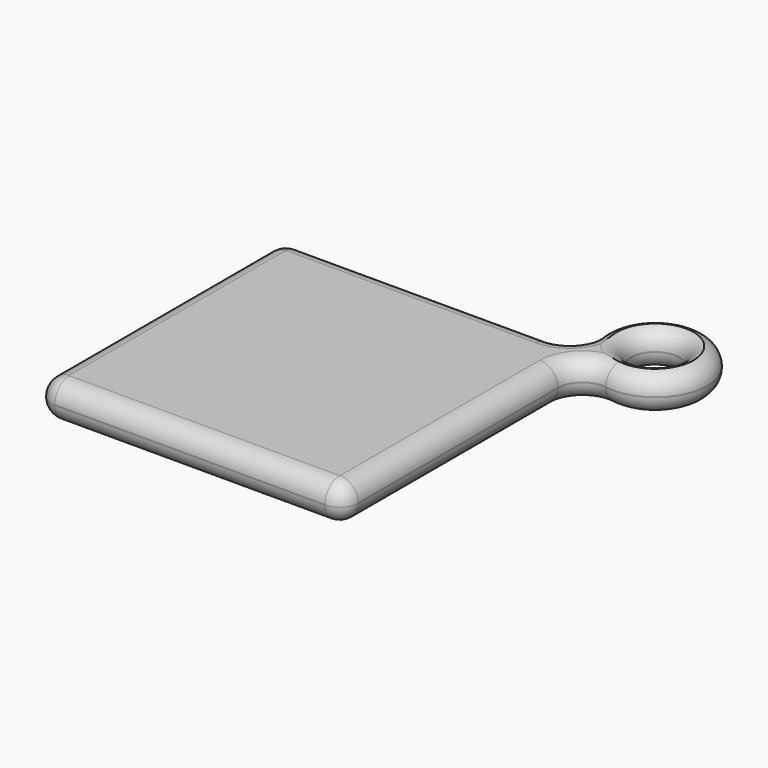
from build123d import *

# Parameters (mm, degrees)
F0_R         = 2
F1_DEPTH     = 3
F2_T1_DEPTH  = 20.3370084506
F2_T3_DEPTH  = 21.9980686292
F2_T5_DEPTH  = 21.9980686292
F2_T7_DEPTH  = 20.3370084506
F2_S11_W     = 1.6515022539
F2_S11_H     = 1.6515022539
F2_T12_DEPTH = 1.651502254
F2_S17_W     = 1.6515022539
F2_S17_H     = 1.6515022539
F2_T18_DEPTH = 1.651502254
F2_S23_W     = 1.6515022539
F2_S23_H     = 1.6515022539
F2_T24_DEPTH = 1.651502254
F2_S29_W     = 1.6515022539
F2_S29_H     = 1.6515022539
F2_T30_DEPTH = 1.651502254
F2_S35_W     = 1.6515022539
F2_S35_H     = 1.6515022539
F2_T36_DEPTH = 1.651502254
F2_S41_W     = 1.6515022539
F2_S41_H     = 1.6515022539
F2_T42_DEPTH = 1.651502254
F2_T46_ANGLE = 99.2178445956
F2_T48_ANGLE = 288.4356891912
F2_T50_ANGLE = 99.2178445956
F2_T54_ANGLE = 99.2178445956
F2_T56_ANGLE = 288.4356891912
F2_T58_ANGLE = 99.2178445956


# Not quite as in the source:
# - a fillet or chamfer that OpenCascade refuses, or shapes differently, is made with other operations: its cross-section is extruded or revolved along the edge and cut away or added


with BuildPart() as f1:
    # F0 (on Top) → F1 (new body)
    with BuildSketch(Plane.XY):
        with BuildLine():
            Line((0, 25), (0, 0))
            Line((0, 0), (25, 0))
            Line((25, 0), (25, 21.837974136))
            ThreePointArc((25, 21.837974136), (25.7039973924, 23.3612525876), (27.320377241, 23.8121469814))
            ThreePointArc((27.320377241, 23.8121469814), (31.7765520504, 26.0666985205), (31, 31))
            ThreePointArc((31, 31), (26.0666985205, 31.7765520504), (23.8121469814, 27.320377241))
            ThreePointArc((23.8121469814, 27.320377241), (23.3612525876, 25.7039973924), (21.837974136, 25))
            Line((21.837974136, 25), (0, 25))
        make_face()
        with Locations((28, 28)):
            Circle(F0_R, mode=Mode.SUBTRACT)
    extrude(amount=F1_DEPTH)

    # F2: fillet of radius 1.5 on 19 edges, made by hand

    # F2_s2 → F2_t1 (cut)
    with BuildSketch(Plane.YZ.offset(1.5009656854)):
        with BuildLine():
            ThreePointArc((25.0004, 1.4990343146), (24.5606601718, 2.5606601718), (23.4990343146, 3.0004))
            Line((23.4990343146, 3.0004), (23.4990343146, 3.1505365685))
            ThreePointArc((23.4990343146, 3.1505365685), (24.2495171573, 3.1501365685), (25, 3.1501365685))
            Line((25, 3.1501365685), (25.1501365685, 3))
            ThreePointArc((25.1501365685, 3), (25.1501365685, 2.2495171573), (25.1505365685, 1.4990343146))
            Line((25.1505365685, 1.4990343146), (25.0004, 1.4990343146))
        make_face()
        with BuildLine():
            ThreePointArc((25.0004, 1.5009656854), (24.5606601718, 0.4393398282), (23.4990343146, -0.0004))
            Line((23.4990343146, -0.0004), (23.4990343146, -0.1505365685))
            ThreePointArc((23.4990343146, -0.1505365685), (24.2495171573, -0.1501365685), (25, -0.1501365685))
            Line((25, -0.1501365685), (25.1501365685, 0))
            ThreePointArc((25.1501365685, 0), (25.1501365685, 0.7504828427), (25.1505365685, 1.5009656854))
            Line((25.1505365685, 1.5009656854), (25.0004, 1.5009656854))
        make_face()
    extrude(amount=F2_T1_DEPTH, mode=Mode.SUBTRACT)

    # F2_s4 → F2_t3 (cut)
    with BuildSketch(Plane.XZ.offset(-23.4990343146)):
        with BuildLine():
            ThreePointArc((1.5009656854, 3.0004), (0.4393398282, 2.5606601718), (-0.0004, 1.4990343146))
            Line((-0.0004, 1.4990343146), (-0.1505365685, 1.4990343146))
            ThreePointArc((-0.1505365685, 1.4990343146), (-0.1501365685, 2.2495171573), (-0.1501365685, 3))
            Line((-0.1501365685, 3), (0, 3.1501365685))
            ThreePointArc((0, 3.1501365685), (0.7504828427, 3.1501365685), (1.5009656854, 3.1505365685))
            Line((1.5009656854, 3.1505365685), (1.5009656854, 3.0004))
        make_face()
        with BuildLine():
            ThreePointArc((1.5009656854, -0.0004), (0.4393398282, 0.4393398282), (-0.0004, 1.5009656854))
            Line((-0.0004, 1.5009656854), (-0.1505365685, 1.5009656854))
            ThreePointArc((-0.1505365685, 1.5009656854), (-0.1501365685, 0.7504828427), (-0.1501365685, 0))
            Line((-0.1501365685, 0), (0, -0.1501365685))
            ThreePointArc((0, -0.1501365685), (0.7504828427, -0.1501365685), (1.5009656854, -0.1505365685))
            Line((1.5009656854, -0.1505365685), (1.5009656854, -0.0004))
        make_face()
    extrude(amount=F2_T3_DEPTH, mode=Mode.SUBTRACT)

    # F2_s6 → F2_t5 (cut)
    with BuildSketch(Plane.YZ.offset(1.5009656854)):
        with BuildLine():
            ThreePointArc((1.5009656854, 3.0004), (0.4393398282, 2.5606601718), (-0.0004, 1.4990343146))
            Line((-0.0004, 1.4990343146), (-0.1505365685, 1.4990343146))
            ThreePointArc((-0.1505365685, 1.4990343146), (-0.1501365685, 2.2495171573), (-0.1501365685, 3))
            Line((-0.1501365685, 3), (0, 3.1501365685))
            ThreePointArc((0, 3.1501365685), (0.7504828427, 3.1501365685), (1.5009656854, 3.1505365685))
            Line((1.5009656854, 3.1505365685), (1.5009656854, 3.0004))
        make_face()
        with BuildLine():
            ThreePointArc((-0.0004, 1.5009656854), (0.4393398282, 0.4393398282), (1.5009656854, -0.0004))
            Line((1.5009656854, -0.0004), (1.5009656854, -0.1505365685))
            ThreePointArc((1.5009656854, -0.1505365685), (0.7504828427, -0.1501365685), (0, -0.1501365685))
            Line((0, -0.1501365685), (-0.1501365685, 0))
            ThreePointArc((-0.1501365685, 0), (-0.1501365685, 0.7504828427), (-0.1505365685, 1.5009656854))
            Line((-0.1505365685, 1.5009656854), (-0.0004, 1.5009656854))
        make_face()
    extrude(amount=F2_T5_DEPTH, mode=Mode.SUBTRACT)

    # F2_s8 → F2_t7 (cut)
    with BuildSketch(Plane.XZ.offset(-21.837974136)):
        with BuildLine():
            ThreePointArc((23.4990343146, 3.0004), (24.5606601718, 2.5606601718), (25.0004, 1.4990343146))
            Line((25.0004, 1.4990343146), (25.1505365685, 1.4990343146))
            ThreePointArc((25.1505365685, 1.4990343146), (25.1501365685, 2.2495171573), (25.1501365685, 3))
            Line((25.1501365685, 3), (25, 3.1501365685))
            ThreePointArc((25, 3.1501365685), (24.2495171573, 3.1501365685), (23.4990343146, 3.1505365685))
            Line((23.4990343146, 3.1505365685), (23.4990343146, 3.0004))
        make_face()
        with BuildLine():
            ThreePointArc((25.0004, 1.5009656854), (24.5606601718, 0.4393398282), (23.4990343146, -0.0004))
            Line((23.4990343146, -0.0004), (23.4990343146, -0.1505365685))
            ThreePointArc((23.4990343146, -0.1505365685), (24.2495171573, -0.1501365685), (25, -0.1501365685))
            Line((25, -0.1501365685), (25.1501365685, 0))
            ThreePointArc((25.1501365685, 0), (25.1501365685, 0.7504828427), (25.1505365685, 1.5009656854))
            Line((25.1505365685, 1.5009656854), (25.0004, 1.5009656854))
        make_face()
    extrude(amount=F2_T7_DEPTH, mode=Mode.SUBTRACT)


with BuildPart() as f2_tool10:
    # F2_s11 → F2_t12 (new body)
    with BuildSketch(Plane.XZ.offset(-23.4990343146)):
        with Locations((0.6752145585, 2.3247854415)):
            Rectangle(F2_S11_W, F2_S11_H)
    extrude(amount=-F2_T12_DEPTH)

    # F2_s13 → F2_t14 (revolve, cut)
    with BuildSketch(Plane(origin=(1.5009656854, 23.4990343146, 1.4990343146), x_dir=(0.7071067812, 0, -0.7071067812), z_dir=(0.7071067812, 0, 0.7071067812))):
        with BuildLine():
            ThreePointArc((0, -1.5013656854), (1.5013656854, 0), (0, 1.5013656854))
            Line((0, 1.5013656854), (0, -1.5013656854))
        make_face()
    revolve(axis=Axis((1.5009656854, 23.4990343146, 1.4990343146), (0, 1, 0)), mode=Mode.SUBTRACT)


with BuildPart() as f1_1:
    add(f1.part)

    # F2_t9: cut F2_tool10
    add(f2_tool10.part, mode=Mode.SUBTRACT)


with BuildPart() as f2_tool16:
    # F2_s17 → F2_t18 (new body)
    with BuildSketch(Plane.YZ.offset(1.5009656854)):
        with Locations((0.6752145585, 2.3247854415)):
            Rectangle(F2_S17_W, F2_S17_H)
    extrude(amount=-F2_T18_DEPTH)

    # F2_s19 → F2_t20 (revolve, cut)
    with BuildSketch(Plane(origin=(1.5009656854, 1.5009656854, 1.4990343146), x_dir=(0, 0.7071067812, -0.7071067812), z_dir=(0, 0.7071067812, 0.7071067812))):
        with BuildLine():
            ThreePointArc((0, -1.5013656854), (1.5013656854, 0), (0, 1.5013656854))
            Line((0, 1.5013656854), (0, -1.5013656854))
        make_face()
    revolve(axis=Axis((1.5009656854, 1.5009656854, 1.4990343146), (-1, 0, 0)), mode=Mode.SUBTRACT)


with BuildPart() as f1_2:
    add(f1_1.part)

    # F2_t15: cut F2_tool16
    add(f2_tool16.part, mode=Mode.SUBTRACT)


with BuildPart() as f2_tool22:
    # F2_s23 → F2_t24 (new body)
    with BuildSketch(Plane.XY.offset(1.4990343146)):
        with Locations((24.3247854415, 0.6752145585)):
            Rectangle(F2_S23_W, F2_S23_H)
    extrude(amount=F2_T24_DEPTH)

    # F2_s25 → F2_t26 (revolve, cut)
    with BuildSketch(Plane(origin=(23.4990343146, 1.5009656854, 1.4990343146), x_dir=(-0.7071067812, 0.7071067812, 0), z_dir=(0.7071067812, 0.7071067812, 0))):
        with BuildLine():
            ThreePointArc((0, -1.5013656854), (1.5013656854, 0), (0, 1.5013656854))
            Line((0, 1.5013656854), (0, -1.5013656854))
        make_face()
    revolve(axis=Axis((23.4990343146, 1.5009656854, 1.4990343146), (0, 0, 1)), mode=Mode.SUBTRACT)


with BuildPart() as f1_3:
    add(f1_2.part)

    # F2_t21: cut F2_tool22
    add(f2_tool22.part, mode=Mode.SUBTRACT)


with BuildPart() as f2_tool28:
    # F2_s29 → F2_t30 (new body)
    with BuildSketch(Plane.XZ.offset(-23.4990343146)):
        with Locations((0.6752145585, 0.6752145585)):
            Rectangle(F2_S29_W, F2_S29_H)
    extrude(amount=-F2_T30_DEPTH)

    # F2_s31 → F2_t32 (revolve, cut)
    with BuildSketch(Plane(origin=(1.5009656854, 23.4990343146, 1.5009656854), x_dir=(0.7071067812, 0, 0.7071067812), z_dir=(-0.7071067812, 0, 0.7071067812))):
        with BuildLine():
            ThreePointArc((0, -1.5013656854), (1.5013656854, 0), (0, 1.5013656854))
            Line((0, 1.5013656854), (0, -1.5013656854))
        make_face()
    revolve(axis=Axis((1.5009656854, 23.4990343146, 1.5009656854), (0, 1, 0)), mode=Mode.SUBTRACT)


with BuildPart() as f1_4:
    add(f1_3.part)

    # F2_t27: cut F2_tool28
    add(f2_tool28.part, mode=Mode.SUBTRACT)


with BuildPart() as f2_tool34:
    # F2_s35 → F2_t36 (new body)
    with BuildSketch(Plane.YZ.offset(1.5009656854)):
        with Locations((0.6752145585, 0.6752145585)):
            Rectangle(F2_S35_W, F2_S35_H)
    extrude(amount=-F2_T36_DEPTH)

    # F2_s37 → F2_t38 (revolve, cut)
    with BuildSketch(Plane(origin=(1.5009656854, 1.5009656854, 1.5009656854), x_dir=(0, 0.7071067812, 0.7071067812), z_dir=(0, -0.7071067812, 0.7071067812))):
        with BuildLine():
            ThreePointArc((0, -1.5013656854), (1.5013656854, 0), (0, 1.5013656854))
            Line((0, 1.5013656854), (0, -1.5013656854))
        make_face()
    revolve(axis=Axis((1.5009656854, 1.5009656854, 1.5009656854), (-1, 0, 0)), mode=Mode.SUBTRACT)


with BuildPart() as f1_5:
    add(f1_4.part)

    # F2_t33: cut F2_tool34
    add(f2_tool34.part, mode=Mode.SUBTRACT)


with BuildPart() as f2_tool40:
    # F2_s41 → F2_t42 (new body)
    with BuildSketch(Plane.YZ.offset(23.4990343146)):
        with Locations((0.6752145585, 0.6752145585)):
            Rectangle(F2_S41_W, F2_S41_H)
    extrude(amount=F2_T42_DEPTH)

    # F2_s43 → F2_t44 (revolve, cut)
    with BuildSketch(Plane(origin=(23.4990343146, 1.5009656854, 1.5009656854), x_dir=(0, 0.7071067812, 0.7071067812), z_dir=(0, 0.7071067812, -0.7071067812))):
        with BuildLine():
            ThreePointArc((0, -1.5013656854), (1.5013656854, 0), (0, 1.5013656854))
            Line((0, 1.5013656854), (0, -1.5013656854))
        make_face()
    revolve(axis=Axis((23.4990343146, 1.5009656854, 1.5009656854), (1, 0, 0)), mode=Mode.SUBTRACT)


with BuildPart() as f1_6:
    add(f1_5.part)

    # F2_t39: cut F2_tool40
    add(f2_tool40.part, mode=Mode.SUBTRACT)

    # F2_s45 → F2_t46 (revolve, cut)
    with BuildSketch(Plane.XZ.offset(-21.837974136)):
        with BuildLine():
            ThreePointArc((23.4990343146, 3.0004), (24.5606601718, 2.5606601718), (25.0004, 1.4990343146))
            Line((25.0004, 1.4990343146), (25.1505365685, 1.4990343146))
            ThreePointArc((25.1505365685, 1.4990343146), (25.1501365685, 2.2495171573), (25.1501365685, 3))
            Line((25.1501365685, 3), (25, 3.1501365685))
            ThreePointArc((25, 3.1501365685), (24.2495171573, 3.1501365685), (23.4990343146, 3.1505365685))
            Line((23.4990343146, 3.1505365685), (23.4990343146, 3.0004))
        make_face()
    revolve(axis=Axis((27, 21.837974136, 3), (0, 0, -1)), revolution_arc=F2_T46_ANGLE, mode=Mode.SUBTRACT)

    # F2_s47 → F2_t48 (revolve, cut)
    with BuildSketch(Plane(origin=(-3.7088693105, 22.8541486176, 0), x_dir=(0, 0, 1), z_dir=(0.1601886205, -0.9870864227, 0))):
        with BuildLine():
            ThreePointArc((3.0004, -29.3820262079), (2.5606601718, -28.3204003507), (1.4990343146, -27.8806605224))
            Line((1.4990343146, -27.8806605224), (1.4990343146, -27.7305239539))
            ThreePointArc((1.4990343146, -27.7305239539), (2.2495171573, -27.7309239539), (3, -27.7309239539))
            Line((3, -27.7309239539), (3.1501365685, -27.8810605224))
            ThreePointArc((3.1501365685, -27.8810605224), (3.1501365685, -28.6315433652), (3.1505365685, -29.3820262079))
            Line((3.1505365685, -29.3820262079), (3.0004, -29.3820262079))
        make_face()
    revolve(axis=Axis((28, 28, 3), (0, 0, -1)), revolution_arc=F2_T48_ANGLE, mode=Mode.SUBTRACT)

    # F2_s49 → F2_t50 (revolve, cut)
    with BuildSketch(Plane(origin=(-3.7088693105, 22.8541486176, 0), x_dir=(0, 0, 1), z_dir=(-0.1601886205, 0.9870864227, 0))):
        with BuildLine():
            ThreePointArc((3.0004, 29.3820262079), (2.5606601718, 28.3204003507), (1.4990343146, 27.8806605224))
            Line((1.4990343146, 27.8806605224), (1.4990343146, 27.7305239539))
            ThreePointArc((1.4990343146, 27.7305239539), (2.2495171573, 27.7309239539), (3, 27.7309239539))
            Line((3, 27.7309239539), (3.1501365685, 27.8810605224))
            ThreePointArc((3.1501365685, 27.8810605224), (3.1501365685, 28.6315433652), (3.1505365685, 29.3820262079))
            Line((3.1505365685, 29.3820262079), (3.0004, 29.3820262079))
        make_face()
    revolve(axis=Axis((21.837974136, 27, 3), (0, 0, -1)), revolution_arc=F2_T50_ANGLE, mode=Mode.SUBTRACT)

    # F2_s51 → F2_t52 (revolve, cut)
    with BuildSketch(Plane.XZ.offset(-28)):
        with BuildLine():
            ThreePointArc((31.5009656854, 3.0004), (30.4393398282, 2.5606601718), (29.9996, 1.4990343146))
            Line((29.9996, 1.4990343146), (29.8494634315, 1.4990343146))
            ThreePointArc((29.8494634315, 1.4990343146), (29.8498634315, 2.2495171573), (29.8498634315, 3))
            Line((29.8498634315, 3), (30, 3.1501365685))
            ThreePointArc((30, 3.1501365685), (30.7504828427, 3.1501365685), (31.5009656854, 3.1505365685))
            Line((31.5009656854, 3.1505365685), (31.5009656854, 3.0004))
        make_face()
    revolve(axis=Axis((28, 28, 3), (0, 0, 1)), mode=Mode.SUBTRACT)

    # F2_s53 → F2_t54 (revolve, cut)
    with BuildSketch(Plane.XZ.offset(-21.837974136)):
        with BuildLine():
            ThreePointArc((25.0004, 1.5009656854), (24.5606601718, 0.4393398282), (23.4990343146, -0.0004))
            Line((23.4990343146, -0.0004), (23.4990343146, -0.1505365685))
            ThreePointArc((23.4990343146, -0.1505365685), (24.2495171573, -0.1501365685), (25, -0.1501365685))
            Line((25, -0.1501365685), (25.1501365685, 0))
            ThreePointArc((25.1501365685, 0), (25.1501365685, 0.7504828427), (25.1505365685, 1.5009656854))
            Line((25.1505365685, 1.5009656854), (25.0004, 1.5009656854))
        make_face()
    revolve(axis=Axis((27, 21.837974136, 0), (0, 0, -1)), revolution_arc=F2_T54_ANGLE, mode=Mode.SUBTRACT)

    # F2_s55 → F2_t56 (revolve, cut)
    with BuildSketch(Plane(origin=(22.8541486176, -3.7088693105, 0), x_dir=(0, 0, 1), z_dir=(-0.9870864227, 0.1601886205, 0))):
        with BuildLine():
            ThreePointArc((1.5009656854, 27.8806605224), (0.4393398282, 28.3204003507), (-0.0004, 29.3820262079))
            Line((-0.0004, 29.3820262079), (-0.1505365685, 29.3820262079))
            ThreePointArc((-0.1505365685, 29.3820262079), (-0.1501365685, 28.6315433652), (-0.1501365685, 27.8810605224))
            Line((-0.1501365685, 27.8810605224), (0, 27.7309239539))
            ThreePointArc((0, 27.7309239539), (0.7504828427, 27.7309239539), (1.5009656854, 27.7305239539))
            Line((1.5009656854, 27.7305239539), (1.5009656854, 27.8806605224))
        make_face()
    revolve(axis=Axis((28, 28, 0), (0, 0, 1)), revolution_arc=F2_T56_ANGLE, mode=Mode.SUBTRACT)

    # F2_s57 → F2_t58 (revolve, cut)
    with BuildSketch(Plane(origin=(-3.7088693105, 22.8541486176, 0), x_dir=(0, 0, 1), z_dir=(-0.1601886205, 0.9870864227, 0))):
        with BuildLine():
            ThreePointArc((-0.0004, 29.3820262079), (0.4393398282, 28.3204003507), (1.5009656854, 27.8806605224))
            Line((1.5009656854, 27.8806605224), (1.5009656854, 27.7305239539))
            ThreePointArc((1.5009656854, 27.7305239539), (0.7504828427, 27.7309239539), (0, 27.7309239539))
            Line((0, 27.7309239539), (-0.1501365685, 27.8810605224))
            ThreePointArc((-0.1501365685, 27.8810605224), (-0.1501365685, 28.6315433652), (-0.1505365685, 29.3820262079))
            Line((-0.1505365685, 29.3820262079), (-0.0004, 29.3820262079))
        make_face()
    revolve(axis=Axis((21.837974136, 27, 0), (0, 0, -1)), revolution_arc=F2_T58_ANGLE, mode=Mode.SUBTRACT)

    # F2_s59 → F2_t60 (revolve, cut)
    with BuildSketch(Plane.XZ.offset(-28)):
        with BuildLine():
            ThreePointArc((29.9996, 1.5009656854), (30.4393398282, 0.4393398282), (31.5009656854, -0.0004))
            Line((31.5009656854, -0.0004), (31.5009656854, -0.1505365685))
            ThreePointArc((31.5009656854, -0.1505365685), (30.7504828427, -0.1501365685), (30, -0.1501365685))
            Line((30, -0.1501365685), (29.8498634315, 0))
            ThreePointArc((29.8498634315, 0), (29.8498634315, 0.7504828427), (29.8494634315, 1.5009656854))
            Line((29.8494634315, 1.5009656854), (29.9996, 1.5009656854))
        make_face()
    revolve(axis=Axis((28, 28, 0), (0, 0, 1)), mode=Mode.SUBTRACT)


solid = f1_6.part
